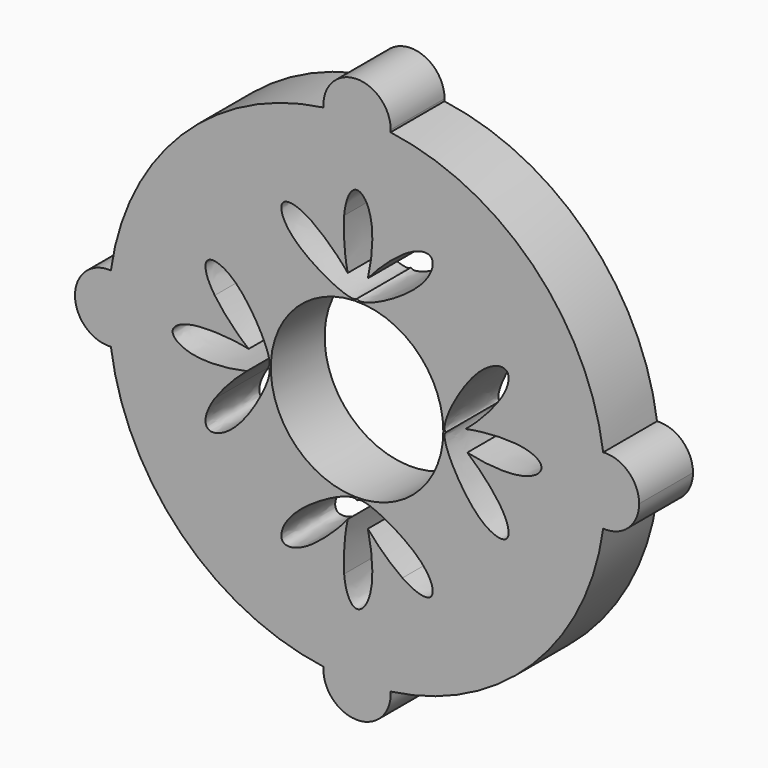
from build123d import *

# Parameters (mm, degrees)
F0_R     = 32.5571544533
F1_DEPTH = 25.4


with BuildPart() as f1:
    # F0 (on Front) → F1 (new body)
    with BuildSketch(Plane.XZ):
        with BuildLine():
            ThreePointArc((72.7026547079, 20.8405979641), (73.3475472363, 27.1614337504), (73.5628410121, 33.5114337504))
            ThreePointArc((73.5628410121, 33.5114337504), (73.3475472363, 39.8614337504), (72.7026547079, 46.1822695366))
            ThreePointArc((72.7026547079, 46.1822695366), (60.8628410121, 33.5114337504), (72.7026547079, 20.8405979641))
        make_face()
        with BuildLine():
            ThreePointArc((72.7026547079, 46.1822695366), (73.3475472363, 39.8614337504), (73.5628410121, 33.5114337504))
            ThreePointArc((73.5628410121, 33.5114337504), (73.3475472363, 27.1614337504), (72.7026547079, 20.8405979641))
            ThreePointArc((72.7026547079, 20.8405979641), (82.2336435682, 24.2320381326), (86.2628410121, 33.5114337504))
            ThreePointArc((86.2628410121, 33.5114337504), (82.2336435682, 42.7908293682), (72.7026547079, 46.1822695366))
        make_face()
        with BuildLine():
            ThreePointArc((72.7026547079, 20.8405979641), (60.8628410121, 33.5114337504), (72.7026547079, 46.1822695366))
            ThreePointArc((72.7026547079, 46.1822695366), (46.1032389276, 99.8047775201), (-7.5192690559, 126.4041933005))
            ThreePointArc((-7.5192690559, 126.4041933005), (-20.1901048422, 114.5643796046), (-32.8609406284, 126.4041933005))
            ThreePointArc((-32.8609406284, 126.4041933005), (-86.4834486119, 99.8047775201), (-113.0828643922, 46.1822695366))
            ThreePointArc((-113.0828643922, 46.1822695366), (-104.6636550786, 42.1822363066), (-101.2430506964, 33.5114337504))
            ThreePointArc((-101.2430506964, 33.5114337504), (-104.6636550786, 24.8406311942), (-113.0828643922, 20.8405979641))
            ThreePointArc((-113.0828643922, 20.8405979641), (-86.4834486119, -32.7819100194), (-32.8609406284, -59.3813257997))
            ThreePointArc((-32.8609406284, -59.3813257997), (-20.1901048422, -47.5415121038), (-7.5192690559, -59.3813257997))
            ThreePointArc((-7.5192690559, -59.3813257997), (46.1032389276, -32.7819100194), (72.7026547079, 20.8405979641))
        make_face()
        with BuildLine():
            add(Edge.make_bspline(
                [(-16.1018727124, -8.0872138884), (-14.8374587809, -13.3588156034), (-13.1205174889, -29.0026812346), (-20.3622985733, -39.9287245765), (-24.4974463507, -32.3981407691), (-25.0515972706, -26.0330624878)],
                knots=[0.4422321589, 0.4422321589, 0.4422321589, 0.4422321589, 0.6004868453, 0.8041385802, 1, 1, 1, 1], degree=3))
            add(Edge.make_bspline(
                [(-25.0515972706, -26.0330624878), (-25.5338579224, -20.4937289052), (-24.9004335132, -12.9297905574), (-23.7030758657, -7.3824363603)],
                knots=[0, 0, 0, 0, 0.1704522226, 0.1704522226, 0.1704522226, 0.1704522226], degree=3))
            add(Edge.make_bspline(
                [(-37.3253126603, -20.1925507096), (-32.7226346039, -17.0729118546), (-27.2525779633, -11.8105102964), (-23.7030758657, -7.3824363603)],
                knots=[0, 0, 0, 0, 0.1704522226, 0.1704522226, 0.1704522226, 0.1704522226], degree=3))
            add(Edge.make_bspline(
                [(-20.1901048422, 0), (-22.0397646286, 2.4253654914), (-46.1688115148, -9.6519237601), (-51.0660045272, -25.3182052214), (-42.6141088114, -23.777232012), (-37.3253126603, -20.1925507096)],
                knots=[0.3015664348, 0.3015664348, 0.3015664348, 0.3015664348, 0.6004868453, 0.8041385802, 1, 1, 1, 1], degree=3))
            add(Edge.make_bspline(
                [(-20.1901048422, 0), (-18.3404450558, 2.4253654914), (5.7886018304, -9.6519237601), (10.6857948428, -25.3182052214), (2.2338991271, -23.777232012), (-3.0548970241, -20.1925507096)],
                knots=[0.3015664348, 0.3015664348, 0.3015664348, 0.3015664348, 0.6004868453, 0.8041385802, 1, 1, 1, 1], degree=3))
            add(Edge.make_bspline(
                [(-3.0548970241, -20.1925507096), (-7.415632291, -17.2368977161), (-12.5549541899, -12.3578327013), (-16.1018727124, -8.0872138884)],
                knots=[0, 0, 0, 0, 0.1614922898, 0.1614922898, 0.1614922898, 0.1614922898], degree=3))
        make_face(mode=Mode.SUBTRACT)
        with BuildLine():
            add(Edge.make_bspline(
                [(-61.788752481, 29.4232016206), (-67.060354196, 28.1587876891), (-82.7042198271, 26.4418463971), (-93.6302631691, 33.6836274815), (-86.0996793616, 37.8187752589), (-79.7346010804, 38.3729261789)],
                knots=[0.4422321589, 0.4422321589, 0.4422321589, 0.4422321589, 0.6004868453, 0.8041385802, 1, 1, 1, 1], degree=3))
            add(Edge.make_bspline(
                [(-79.7346010804, 38.3729261789), (-74.1952674978, 38.8551868307), (-66.63132915, 38.2217624214), (-61.0839749529, 37.0244047739)],
                knots=[0, 0, 0, 0, 0.1704522226, 0.1704522226, 0.1704522226, 0.1704522226], degree=3))
            add(Edge.make_bspline(
                [(-73.8940893022, 50.6466415685), (-70.7744504472, 46.0439635121), (-65.512048889, 40.5739068715), (-61.0839749529, 37.0244047739)],
                knots=[0, 0, 0, 0, 0.1704522226, 0.1704522226, 0.1704522226, 0.1704522226], degree=3))
            add(Edge.make_bspline(
                [(-53.7015385926, 33.5114337504), (-51.2761731011, 35.3610935368), (-63.3534623526, 59.490140423), (-79.0197438139, 64.3873334354), (-77.4787706045, 55.9354377196), (-73.8940893022, 50.6466415685)],
                knots=[0.3015664348, 0.3015664348, 0.3015664348, 0.3015664348, 0.6004868453, 0.8041385802, 1, 1, 1, 1], degree=3))
            add(Edge.make_bspline(
                [(-53.7015385926, 33.5114337504), (-51.2761731011, 31.661773964), (-63.3534623526, 7.5327270778), (-79.0197438139, 2.6355340654), (-77.4787706045, 11.0874297811), (-73.8940893022, 16.3762259323)],
                knots=[0.3015664348, 0.3015664348, 0.3015664348, 0.3015664348, 0.6004868453, 0.8041385802, 1, 1, 1, 1], degree=3))
            add(Edge.make_bspline(
                [(-73.8940893022, 16.3762259323), (-70.9384363087, 20.7369611992), (-66.0593712938, 25.8762830981), (-61.788752481, 29.4232016206)],
                knots=[0, 0, 0, 0, 0.1614922898, 0.1614922898, 0.1614922898, 0.1614922898], degree=3))
        make_face(mode=Mode.SUBTRACT)
        with Locations((-20.1901048422, 33.5114337504)):
            Circle(F0_R, mode=Mode.SUBTRACT)
        with BuildLine():
            add(Edge.make_bspline(
                [(39.354391396, 38.3729261789), (33.8150578134, 38.8551868307), (26.2511194656, 38.2217624214), (20.7037652685, 37.0244047739)],
                knots=[0, 0, 0, 0, 0.1704522226, 0.1704522226, 0.1704522226, 0.1704522226], degree=3))
            add(Edge.make_bspline(
                [(21.4085427966, 29.4232016206), (26.6801445116, 28.1587876891), (42.3240101428, 26.4418463971), (53.2500534847, 33.6836274815), (45.7194696773, 37.8187752589), (39.354391396, 38.3729261789)],
                knots=[0.4422321589, 0.4422321589, 0.4422321589, 0.4422321589, 0.6004868453, 0.8041385802, 1, 1, 1, 1], degree=3))
            add(Edge.make_bspline(
                [(33.5138796178, 16.3762259323), (30.5582266244, 20.7369611992), (25.6791616095, 25.8762830981), (21.4085427966, 29.4232016206)],
                knots=[0, 0, 0, 0, 0.1614922898, 0.1614922898, 0.1614922898, 0.1614922898], degree=3))
            add(Edge.make_bspline(
                [(13.3213289082, 33.5114337504), (10.8959634168, 31.661773964), (22.9732526683, 7.5327270778), (38.6395341296, 2.6355340654), (37.0985609202, 11.0874297811), (33.5138796178, 16.3762259323)],
                knots=[0.3015664348, 0.3015664348, 0.3015664348, 0.3015664348, 0.6004868453, 0.8041385802, 1, 1, 1, 1], degree=3))
            add(Edge.make_bspline(
                [(13.3213289082, 33.5114337504), (10.8959634168, 35.3610935368), (22.9732526683, 59.490140423), (38.6395341296, 64.3873334354), (37.0985609202, 55.9354377196), (33.5138796178, 50.6466415685)],
                knots=[0.3015664348, 0.3015664348, 0.3015664348, 0.3015664348, 0.6004868453, 0.8041385802, 1, 1, 1, 1], degree=3))
            add(Edge.make_bspline(
                [(33.5138796178, 50.6466415685), (30.3942407628, 46.0439635122), (25.1318392046, 40.5739068715), (20.7037652685, 37.0244047739)],
                knots=[0, 0, 0, 0, 0.1704522226, 0.1704522226, 0.1704522226, 0.1704522226], degree=3))
        make_face(mode=Mode.SUBTRACT)
        with BuildLine():
            add(Edge.make_bspline(
                [(-25.0515972706, 93.0559299886), (-25.5338579224, 87.516596406), (-24.9004335132, 79.9526580582), (-23.7030758657, 74.4053038611)],
                knots=[0, 0, 0, 0, 0.1704522226, 0.1704522226, 0.1704522226, 0.1704522226], degree=3))
            add(Edge.make_bspline(
                [(-16.1018727124, 75.1100813892), (-14.8374587809, 80.3816831042), (-13.1205174889, 96.0255487353), (-20.3622985733, 106.9515920773), (-24.4974463507, 99.4210082698), (-25.0515972706, 93.0559299886)],
                knots=[0.4422321589, 0.4422321589, 0.4422321589, 0.4422321589, 0.6004868453, 0.8041385802, 1, 1, 1, 1], degree=3))
            add(Edge.make_bspline(
                [(-3.0548970241, 87.2154182104), (-7.415632291, 84.2597652169), (-12.5549541899, 79.380700202), (-16.1018727124, 75.1100813892)],
                knots=[0, 0, 0, 0, 0.1614922898, 0.1614922898, 0.1614922898, 0.1614922898], degree=3))
            add(Edge.make_bspline(
                [(7.3836464649, 84.3488277478), (8.5684994899, 86.7406655992), (8.8730403963, 92.0105662735), (2.2338991271, 90.8000995127), (-3.0548970241, 87.2154182104)],
                knots=[0.6861740416, 0.6861740416, 0.6861740416, 0.6861740416, 0.8041385802, 1, 1, 1, 1], degree=3))
            add(Edge.make_bspline(
                [(7.3836464648, 84.348827748), (10.0527060203, 84.3785949738), (14.9328812478, 82.3665094814), (10.9617364962, 76.9100054786), (5.437364977, 73.7002353798)],
                knots=[0.6861740416, 0.6861740416, 0.6861740416, 0.6861740416, 0.8041385802, 1, 1, 1, 1], degree=3))
            add(Edge.make_bspline(
                [(5.437364977, 73.7002353798), (-3.0684705553, 68.7581751904), (-18.7951923439, 64.2800044612), (-20.1901048422, 67.0228675008)],
                knots=[0, 0, 0, 0, 0.3015664348, 0.3015664348, 0.3015664348, 0.3015664348], degree=3))
            add(Edge.make_bspline(
                [(-20.1901048422, 67.0228675008), (-22.0397646286, 64.5975020093), (-46.1688115148, 76.6747912609), (-51.0660045272, 92.3410727222), (-42.6141088114, 90.8000995127), (-37.3253126603, 87.2154182104)],
                knots=[0.3015664348, 0.3015664348, 0.3015664348, 0.3015664348, 0.6004868453, 0.8041385802, 1, 1, 1, 1], degree=3))
            add(Edge.make_bspline(
                [(-37.3253126603, 87.2154182104), (-32.7226346039, 84.0957793554), (-27.2525779633, 78.8333777972), (-23.7030758657, 74.4053038611)],
                knots=[0, 0, 0, 0, 0.1704522226, 0.1704522226, 0.1704522226, 0.1704522226], degree=3))
        make_face(mode=Mode.SUBTRACT)
        with BuildLine():
            ThreePointArc((-32.8609406284, 126.4041933005), (-20.1901048422, 114.5643796046), (-7.5192690559, 126.4041933005))
            ThreePointArc((-7.5192690559, 126.4041933005), (-20.1901048422, 127.2643796046), (-32.8609406284, 126.4041933005))
        make_face()
        with BuildLine():
            ThreePointArc((-32.8609406284, 126.4041933005), (-20.1901048422, 127.2643796046), (-7.5192690559, 126.4041933005))
            ThreePointArc((-7.5192690559, 126.4041933005), (-7.4973979897, 126.8340393238), (-7.4901048422, 127.2643796046))
            ThreePointArc((-7.4901048422, 127.2643796046), (-20.620445123, 139.9570864571), (-32.8609406284, 126.4041933005))
        make_face()
        with BuildLine():
            ThreePointArc((-7.4901048422, -60.2415121038), (-7.4973979897, -59.811171823), (-7.5192690559, -59.3813257997))
            ThreePointArc((-7.5192690559, -59.3813257997), (-20.1901048422, -60.2415121038), (-32.8609406284, -59.3813257997))
            ThreePointArc((-32.8609406284, -59.3813257997), (-20.620445123, -72.9342189563), (-7.4901048422, -60.2415121038))
        make_face()
        with BuildLine():
            ThreePointArc((-32.8609406284, -59.3813257997), (-20.1901048422, -60.2415121038), (-7.5192690559, -59.3813257997))
            ThreePointArc((-7.5192690559, -59.3813257997), (-20.1901048422, -47.5415121038), (-32.8609406284, -59.3813257997))
        make_face()
        with BuildLine():
            ThreePointArc((-101.2430506964, 33.5114337504), (-104.6636550786, 42.1822363066), (-113.0828643922, 46.1822695366))
            ThreePointArc((-113.0828643922, 46.1822695366), (-113.9430506964, 33.5114337504), (-113.0828643922, 20.8405979641))
            ThreePointArc((-113.0828643922, 20.8405979641), (-104.6636550786, 24.8406311942), (-101.2430506964, 33.5114337504))
        make_face()
        with BuildLine():
            ThreePointArc((-113.0828643922, 20.8405979641), (-113.9430506964, 33.5114337504), (-113.0828643922, 46.1822695366))
            ThreePointArc((-113.0828643922, 46.1822695366), (-126.6430506964, 33.5114337504), (-113.0828643922, 20.8405979641))
        make_face()
        with BuildLine():
            add(Edge.make_bspline(
                [(-20.1901048422, 67.0228675008), (-18.3404450558, 64.5975020093), (0.1249933138, 73.8399905916), (6.5229917716, 82.6114422419), (7.3836464649, 84.3488277478)],
                knots=[0.3015664348, 0.3015664348, 0.3015664348, 0.3015664348, 0.6004868453, 0.6861740416, 0.6861740416, 0.6861740416, 0.6861740416], degree=3))
            add(Edge.make_bspline(
                [(5.437364977, 73.7002353798), (-3.0684705553, 68.7581751904), (-18.7951923439, 64.2800044612), (-20.1901048422, 67.0228675008)],
                knots=[0, 0, 0, 0, 0.3015664348, 0.3015664348, 0.3015664348, 0.3015664348], degree=3))
            add(Edge.make_bspline(
                [(7.3836464648, 84.348827748), (10.0527060203, 84.3785949738), (14.9328812478, 82.3665094814), (10.9617364962, 76.9100054786), (5.437364977, 73.7002353798)],
                knots=[0.6861740416, 0.6861740416, 0.6861740416, 0.6861740416, 0.8041385802, 1, 1, 1, 1], degree=3))
        make_face()
    extrude(amount=F1_DEPTH)


solid = f1.part
